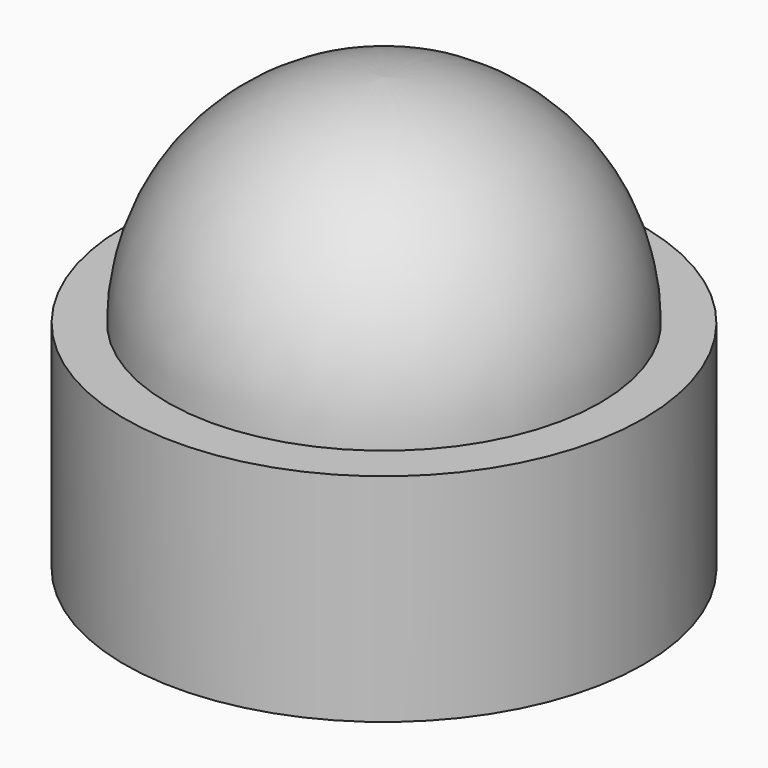
from build123d import *

# Parameters (mm, degrees)
F0_R     = 6
F1_DEPTH = 5
F3_R     = 5
F4_DEPTH = 5
F5_R     = 4.99999


# Not quite as in the source:
# - a fillet or chamfer is up to 0.001 mm smaller than in the source, because OpenCascade refuses the exact size


with BuildPart() as f1:
    # F0 (on Top) → F1 (new body)
    with BuildSketch(Plane.XY):
        Circle(F0_R)
    extrude(amount=F1_DEPTH)

    # F3 (on face) → F4 (join)
    with BuildSketch(Plane.XY.offset(5)):
        Circle(F3_R)
    extrude(amount=F4_DEPTH)

    # F5 (radius 5 in the source; OpenCascade refuses exactly that, so slightly less here)
    f5_edges = [f1.edges().sort_by_distance(p)[0] for p in [
        (-5, 0, 10),
    ]]
    fillet(f5_edges, radius=F5_R)


solid = f1.part
